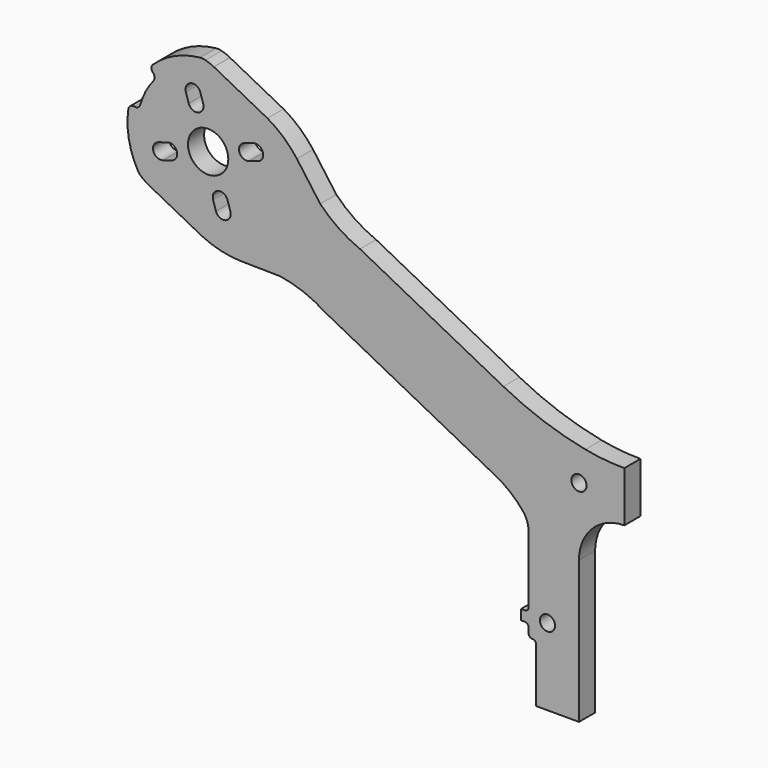
from build123d import *

# Parameters (mm, degrees)
F0_R     = 1.5
F0_R_2   = 4
F1_DEPTH = 4


# Not quite as in the source:
# - ends of sketch curves that miss each other by under 0.0002 mm in the source are joined


with BuildPart() as f1:
    # F0 (on Front) → F1 (new body)
    with BuildSketch(Plane.XZ):
        with BuildLine():
            ThreePointArc((-46.7520374748, 33.7019691352), (-47.1985525616, 33.1188473182), (-47.9229891353, 32.9980233677))
            ThreePointArc((-47.9229891353, 32.9980233677), (-48.7034151976, 32.8409436846), (-49.1218329373, 32.1636949909))
            ThreePointArc((-49.1218329373, 32.1636949909), (-49.0191167234, 26.9485703376), (-47.2444231086, 22.0436199391))
            ThreePointArc((-47.2444231086, 22.0436199391), (-46.9316892388, 21.5893722277), (-46.5410881725, 21.2000467918))
            ThreePointArc((-46.5410881725, 21.2000467918), (-45.835088561, 20.6717193883), (-45.0805279455, 20.2154261011))
            ThreePointArc((-45.0805279455, 20.2154261011), (-45.0596673609, 20.2042820611), (-45.0387197194, 20.1933025406))
            Line((-45.0387197194, 20.1933025406), (-34.428702, 14.685356))
            ThreePointArc((-34.428702, 14.685356), (-30.7249663127, 13.3838083991), (-26.831855016, 12.8784683528))
            Line((-26.831855016, 12.8784683528), (-18.940113, 12.75863))
            ThreePointArc((-18.940113, 12.75863), (-14.3281771728, 11.5292251091), (-10.0737090286, 9.3656889559))
            Line((-10.0737090286, 9.3656889559), (23.742856, -8.189399))
            ThreePointArc((23.742856, -8.189399), (26.6741197813, -10.1115239367), (29.157366832, -12.5854591375))
            ThreePointArc((29.157366832, -12.5854591375), (29.9965212655, -14.0706922033), (30.287531, -15.751588))
            Line((30.287531, -15.751588), (30.287531, -29.049112))
            ThreePointArc((30.287531, -29.049112), (30.0678610859, -29.5794420859), (29.537531, -29.799112))
            Line((29.537531, -29.799112), (28.787531, -29.799112))
            Line((28.787531, -29.799112), (28.787531, -31.799112))
            Line((28.787531, -31.799112), (29.537531, -31.799112))
            ThreePointArc((29.537531, -31.799112), (30.0678610859, -32.0187819141), (30.287531, -32.549112))
            Line((30.287531, -32.549112), (30.287531, -33.549112))
            ThreePointArc((30.287531, -33.549112), (30.5072009141, -34.0794420859), (31.037531, -34.299112))
            ThreePointArc((31.037531, -34.299112), (31.5678610859, -34.5187819141), (31.787531, -35.049112))
            Line((31.787531, -35.049112), (31.787531, -45.799112))
            Line((31.787531, -45.799112), (40.287531, -45.799112))
            Line((40.287531, -45.799112), (40.287531, -17.549112))
            ThreePointArc((40.287531, -17.549112), (42.9235699693, -11.1851509693), (49.287531, -8.549112))
            Line((49.287531, -8.549112), (49.287531, 1.450888))
            ThreePointArc((49.287531, 1.450888), (45.4037577728, 1.6406387059), (41.5569790733, 2.2080833707))
            ThreePointArc((41.5569790733, 2.2080833707), (33.2204107171, 4.4808989987), (25.2886487268, 7.9089034738))
            Line((25.2886487268, 7.9089034738), (-3.162569, 22.678696))
            ThreePointArc((-3.162569, 22.678696), (-7.380174163, 24.9132414841), (-11.0394989374, 27.9776710605))
            Line((-11.0394989374, 27.9776710605), (-15.678673, 34.362967))
            ThreePointArc((-15.678673, 34.362967), (-18.332187349, 37.2561568684), (-21.5279068846, 39.5363022038))
            Line((-21.5279068846, 39.5363022038), (-32.137926, 45.044248))
            ThreePointArc((-32.137926, 45.044248), (-32.1589591581, 45.0550621571), (-32.1800770412, 45.0657099174))
            ThreePointArc((-32.1800770412, 45.0657099174), (-32.9874548739, 45.4202604433), (-33.8258020362, 45.693644867))
            ThreePointArc((-33.8258020362, 45.693644867), (-34.3689763365, 45.7890671015), (-34.9204399653, 45.7834476614))
            ThreePointArc((-34.9204399653, 45.7834476614), (-39.9164421929, 44.4291859973), (-44.218633855, 41.550781845))
            ThreePointArc((-44.218633855, 41.550781845), (-44.5354399962, 40.8204576148), (-44.2185063254, 40.090188652))
            ThreePointArc((-44.2185063254, 40.090188652), (-43.903802542, 39.4265860913), (-44.1273026907, 38.7269757472))
            ThreePointArc((-44.1273026907, 38.7269757472), (-45.6966868361, 36.3487212178), (-46.7520374748, 33.7019691352))
        make_face()
        with Locations((34.037531, -30.549112)):
            Circle(F0_R, mode=Mode.SUBTRACT)
        with Locations((40.287531, -4.049112)):
            Circle(F0_R, mode=Mode.SUBTRACT)
        with BuildLine():
            Line((-29.443172, 22.692668), (-28.872421, 20.889608))
            ThreePointArc((-28.872421, 20.889608), (-29.8498040801, 19.0068647531), (-31.7325472924, 19.984248224))
            Line((-31.7325472924, 19.984248224), (-32.303298, 21.787307))
            ThreePointArc((-32.303298, 21.787307), (-31.3259155182, 23.6700510575), (-29.443172, 22.692668))
        make_face(mode=Mode.SUBTRACT)
        with BuildLine():
            Line((-40.461853, 26.022633), (-42.264913, 25.451882))
            ThreePointArc((-42.264913, 25.451882), (-44.1476570575, 26.4292644818), (-43.1702740637, 28.3120082014))
            Line((-43.1702740637, 28.3120082014), (-41.367214, 28.882759))
            ThreePointArc((-41.367214, 28.882759), (-39.4844709425, 27.9053765182), (-40.461853, 26.022633))
        make_face(mode=Mode.SUBTRACT)
        with Locations((-33.28753, 29.866991)):
            Circle(F0_R_2, mode=Mode.SUBTRACT)
        with BuildLine():
            Line((-26.113207, 33.711349), (-24.310148, 34.2821))
            ThreePointArc((-24.310148, 34.2821), (-22.4274039425, 33.3047175182), (-23.4047869363, 31.4219737986))
            Line((-23.4047869363, 31.4219737986), (-25.207847, 30.851223))
            ThreePointArc((-25.207847, 30.851223), (-27.0905902014, 31.8286059363), (-26.113207, 33.711349))
        make_face(mode=Mode.SUBTRACT)
        with BuildLine():
            Line((-37.131889, 37.041314), (-37.70264, 38.844374))
            ThreePointArc((-37.70264, 38.844374), (-36.7252563743, 40.727117103), (-34.8425130864, 39.7497349727))
            Line((-34.8425130864, 39.7497349727), (-34.271762, 37.946675))
            ThreePointArc((-34.271762, 37.946675), (-35.2491456257, 36.063930897), (-37.131889, 37.041314))
        make_face(mode=Mode.SUBTRACT)
    extrude(amount=F1_DEPTH)


solid = f1.part
